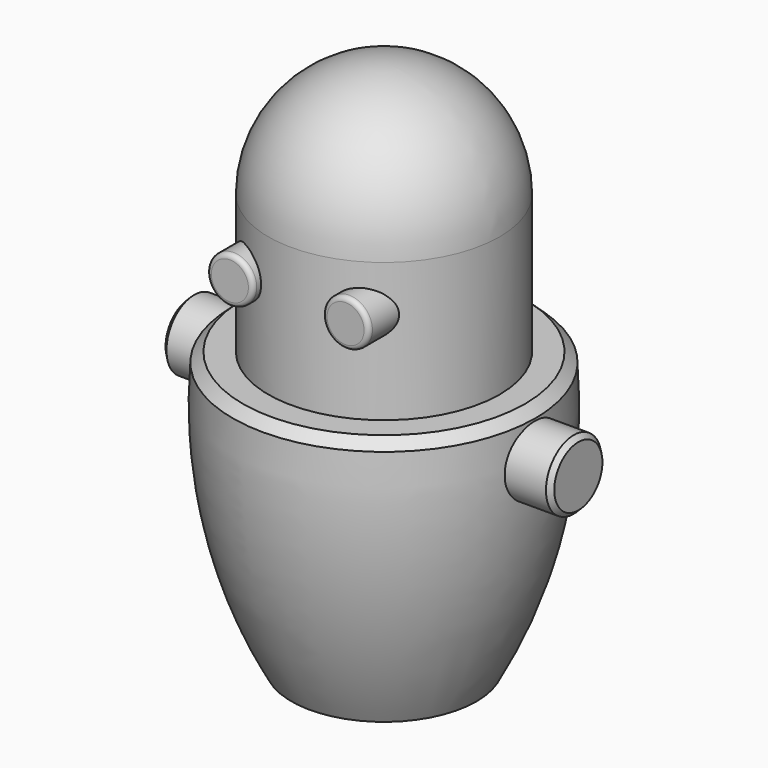
from build123d import *

# Parameters (mm, degrees)
F3_R      = 25
F5_DEPTH  = 55
F6_R      = 25
F4_R      = 5
F7_DEPTH  = 26
F10_DEPTH = 42
F11_SIZE  = 1


# Not quite as in the source:
# - a fillet or chamfer that OpenCascade refuses, or shapes differently, is made with other operations: its cross-section is extruded or revolved along the edge and cut away or added


with BuildPart() as f1:
    # F0 (on Front) → F1 (revolve)
    with BuildSketch(Plane.XZ):
        with BuildLine():
            Line((0, 60), (0, 0))
            Line((0, 0), (20, 0))
            ThreePointArc((20, 0), (30.7804742264, 29.0561512028), (32.5, 60))
            Line((32.5, 60), (0, 60))
        make_face()
    revolve(axis=Axis((0, 0, 30), (0, 0, 1)))

    # F2: chamfer of 2 on 1 edges, made by hand

    # F2_s1 → F2_t2 (revolve, cut)
    with BuildSketch(Plane.XZ):
        with BuildLine():
            Line((30.42161571, 60.0544167929), (32.7310120298, 57.9113922058))
            Line((32.7310120298, 57.9113922058), (32.7709004847, 57.914377364))
            ThreePointArc((32.7709004847, 57.914377364), (32.6335391575, 58.9572189948), (32.539822014, 60.0037692442))
            Line((32.539822014, 60.0037692442), (32.5, 60.04))
            ThreePointArc((32.5, 60.04), (31.460807855, 60.04), (30.42161571, 60.0944167929))
            Line((30.42161571, 60.0944167929), (30.42161571, 60.0544167929))
        make_face()
    revolve(axis=Axis((0, 0, 60), (0, 0, 1)), mode=Mode.SUBTRACT)


with BuildPart() as f5:
    # F3 (on face) → F5 (new body)
    with BuildSketch(Plane.XY.offset(60)):
        Circle(F3_R)
    extrude(amount=F5_DEPTH)

    # F6
    f6_edges = [f5.edges().sort_by_distance(p)[0] for p in [
        (-25, 0, 115),
    ]]
    fillet(f6_edges, radius=F6_R)


with BuildPart() as f7:
    # F4 (on Front) → F7 (new body)
    with BuildSketch(Plane.XZ):
        with Locations((-12.5, 80)):
            Circle(F4_R)
    extrude(amount=F7_DEPTH)

    # F8: fillet of radius 1 on 1 edges, made by hand

    # F8_s1 → F8_t2 (revolve, cut)
    with BuildSketch(Plane.XY.offset(80)):
        with BuildLine():
            ThreePointArc((-7.5, -25), (-7.7928932188, -25.7071067812), (-8.5, -26))
            Line((-8.5, -26), (-7.5, -26))
            Line((-7.5, -26), (-7.5, -25))
        make_face()
    revolve(axis=Axis((-12.5, -26, 80), (0, -1, 0)), mode=Mode.SUBTRACT)


with BuildPart() as f7b:
    # F4 (on Front) → F7, piece 2 (new body)
    with BuildSketch(Plane.XZ):
        with BuildLine():
            ThreePointArc((17.5, 80), (12.5, 85), (7.5, 80))
            ThreePointArc((7.5, 80), (12.5, 75), (17.5, 80))
        make_face()
    extrude(amount=F7_DEPTH)

    # F8#2: fillet of radius 1 on 1 edges, made by hand

    # F8_2_s1 → F8_2_t2 (revolve, cut)
    with BuildSketch(Plane.XY.offset(80)):
        with BuildLine():
            ThreePointArc((17.5, -25), (17.2071067812, -25.7071067812), (16.5, -26))
            Line((16.5, -26), (17.5, -26))
            Line((17.5, -26), (17.5, -25))
        make_face()
    revolve(axis=Axis((12.5, -26, 80), (0, 1, 0)), mode=Mode.SUBTRACT)


with BuildPart() as f10:
    # F9 (on Right) → F10 (new body, symmetric)
    with BuildSketch(Plane.YZ):
        with BuildLine():
            ThreePointArc((0, 42.5), (5.3033008589, 44.6966991411), (7.5, 50))
            ThreePointArc((7.5, 50), (-5.3033008589, 55.3033008589), (0, 42.5))
        make_face()
    extrude(amount=F10_DEPTH, both=True)

    # F11
    f11_edges = [f10.edges().sort_by_distance(p)[0] for p in [
        (42, -5.303301, 55.303301),
        (-42, -5.303301, 55.303301),
        (-42, 5.303301, 44.696699),
        (42, 5.303301, 44.696699),
    ]]
    chamfer(f11_edges, length=F11_SIZE)


solid = Compound([f1.part, f5.part, f7.part, f7b.part, f10.part])
